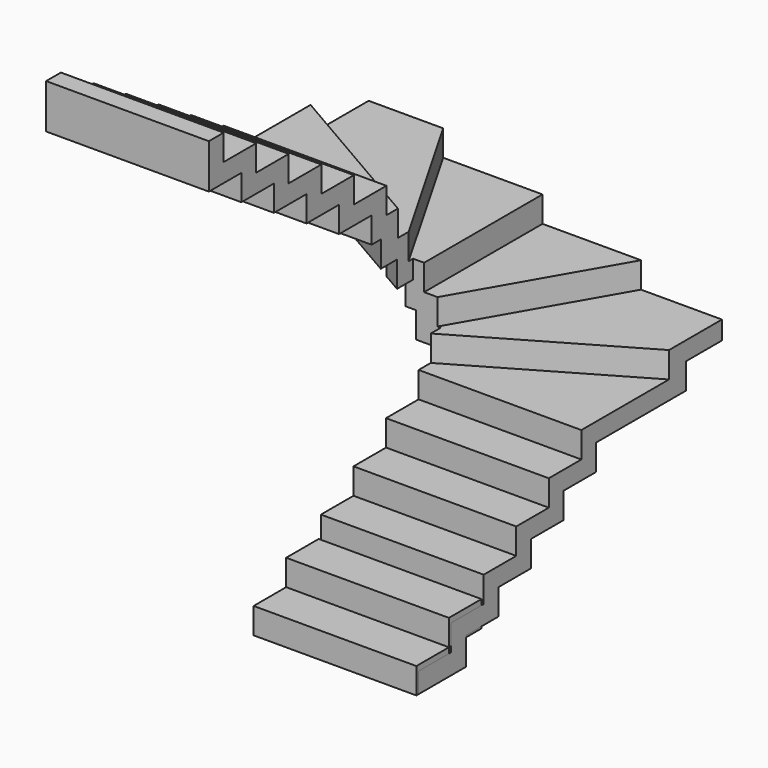
from build123d import *

# Parameters (mm, degrees)
F4_W           = 1117.6
F4_H           = 279.4
F6_DEPTH       = 177.8
F7_START       = 177.8
F7_DEPTH       = 177.8
F8_W           = 260.35
F8_H           = 139.7
F9_DEPTH       = 1117.6
F11_DEPTH      = 127
F12_DEPTH      = 177.8
F12_DEPTH_BACK = 127
F14_DEPTH      = 127
F15_DEPTH      = 177.8
F15_DEPTH_BACK = 127
F17_DEPTH      = 127
F18_DEPTH      = 177.8
F18_DEPTH_BACK = 127
F20_DEPTH      = 127
F21_DEPTH      = 177.8
F21_DEPTH_BACK = 127
F23_DEPTH      = 127
F24_DEPTH      = 177.8
F24_DEPTH_BACK = 127
F26_DEPTH      = 127
F27_DEPTH      = 177.8
F27_DEPTH_BACK = 127
F29_DEPTH      = 1117.6
F31_DEPTH      = 177.8


# Not quite as in the source:
# - a variable given as a bare number and used for a length is read in inches; the dataset says mm whatever the document's units were
# - a feature names something its author has since deleted; it is built from what else it names


with BuildPart() as f6:
    # F4 (on Top) → F6 (new body)
    with BuildSketch(Plane.XY):
        with Locations((654.05, -1257.3)):
            Rectangle(F4_W, F4_H)
    extrude(amount=F6_DEPTH)


with BuildPart() as f7:
    # F4 (on Top) → F7 (new body)
    with BuildSketch(Plane.XY.offset(F7_START)):
        with Locations((654.05, -977.9)):
            Rectangle(F4_W, F4_H)
    extrude(amount=F7_DEPTH)


with BuildPart() as f9:
    # F8 (on face) → F9 (new body)
    with BuildSketch(Plane.YZ.offset(1212.85)):
        Polygon((-1098.55, 139.7), (-1117.6, 139.7), (-1117.6, 0), (-971.55, 0), (-971.55, 190.5), (-692.15, 190.5), (-692.15, 368.3), (-412.75, 368.3), (-412.75, 546.1), (-133.35, 546.1), (-133.35, 723.9), (146.05, 723.9), (146.05, 1028.7), (19.05, 1028.7), (19.05, 850.9), (-260.35, 850.9), (-260.35, 673.1), (-539.75, 673.1), (-539.75, 495.3), (-819.15, 495.3), (-819.15, 317.5), (-1098.55, 317.5), align=None)
        with Locations((-1247.775, 69.85)):
            Rectangle(F8_W, F8_H)
    extrude(amount=-F9_DEPTH)

    # F10 (on face) → F11 (join)
    with BuildSketch(Plane.XY.offset(1028.7)):
        Polygon((1212.85, 771.3179841809), (133.9562233742, 146.05), (1212.85, 146.05), align=None)
    extrude(amount=-F11_DEPTH)

    # F10 (on face) → F12 (join, two sides)
    with BuildSketch(Plane.XY.offset(1028.7)) as f12_sk:
        Polygon((95.25, 146.05), (133.9562233742, 146.05), (1212.85, 771.3179841809), (1212.85, 918.1045453867), (-9.7539214515, 209.55), (95.25, 209.55), align=None)
        Polygon((95.25, 146.05), (95.25, 123.6179841809), (133.9562233742, 146.05), align=None)
    extrude(amount=F12_DEPTH)
    extrude(f12_sk.sketch, amount=-F12_DEPTH_BACK)

    # F13 (on face) → F14 (join)
    with BuildSketch(Plane.XY.offset(1206.5)):
        Polygon((1212.85, 1225.55), (657.4753068494, 1225.55), (114.7722326257, 281.7185665675), (1212.85, 918.1045453867), align=None)
    extrude(amount=-F14_DEPTH)

    # F13 (on face) → F15 (join, two sides)
    with BuildSketch(Plane.XY.offset(1206.5)) as f15_sk:
        Polygon((657.4753068494, 1225.55), (510.9773525122, 1225.55), (-73.2226474878, 209.55), (-9.7539214515, 209.55), (114.7722326257, 281.7185665675), align=None)
        Polygon((114.7722326257, 281.7185665675), (-9.7539214515, 209.55), (73.2753068494, 209.55), align=None)
    extrude(amount=F15_DEPTH)
    extrude(f15_sk.sketch, amount=-F15_DEPTH_BACK)

    # F16 (on face) → F17 (join)
    with BuildSketch(Plane.XY.offset(1384.3)):
        Polygon((510.9773525122, 1225.55), (-19.05, 1225.55), (-19.05, 303.7632999789), align=None)
    extrude(amount=-F17_DEPTH)

    # F16 (on face) → F18 (join, two sides)
    with BuildSketch(Plane.XY.offset(1384.3)) as f18_sk:
        Polygon((-19.05, 1225.55), (-146.05, 1225.55), (-146.05, 209.55), (-73.2226474878, 209.55), (-19.05, 303.7632999789), align=None)
        Polygon((-19.05, 303.7632999789), (-73.2226474878, 209.55), (-19.05, 209.55), align=None)
    extrude(amount=F18_DEPTH)
    extrude(f18_sk.sketch, amount=-F18_DEPTH_BACK)

    # F19 (on face) → F20 (join)
    with BuildSketch(Plane.XY.offset(1562.1)):
        Polygon((-146.05, 1225.55), (-701.4246931506, 1225.55), (-146.05, 259.6809684338), align=None)
        Polygon((-95.25, 209.55), (-117.2246931506, 209.55), (-95.25, 171.3331423468), align=None)
    extrude(amount=-F20_DEPTH)

    # F19 (on face) → F21 (join, two sides)
    with BuildSketch(Plane.XY.offset(1562.1)) as f21_sk:
        Polygon((-146.05, 259.6809684338), (-701.4246931506, 1225.55), (-847.9226474878, 1225.55), (-229.5123430682, 150.0538184006), (-95.25, 72.2426877588), (-95.25, 171.3331423468), (-117.2246931506, 209.55), (-146.05, 209.55), align=None)
        Polygon((-117.2246931506, 209.55), (-146.05, 259.6809684338), (-146.05, 209.55), align=None)
    extrude(amount=F21_DEPTH)
    extrude(f21_sk.sketch, amount=-F21_DEPTH_BACK)

    # F22 (on face) → F23 (join)
    with BuildSketch(Plane.XY.offset(1739.9)):
        Polygon((-235.841614476, 161.0612469359), (-847.9226474878, 1225.55), (-1212.85, 1225.55), (-1212.85, 727.2820158191), align=None)
    extrude(amount=-F23_DEPTH)

    # F22 (on face) → F24 (join, two sides)
    with BuildSketch(Plane.XY.offset(1739.9)) as f24_sk:
        Polygon((-229.5123430682, 150.0538184006), (-235.841614476, 161.0612469359), (-1212.85, 727.2820158191), (-1212.85, 580.4954546133), (-95.25, -67.2045453867), (-95.25, 72.2426877588), align=None)
        Polygon((-95.25, 79.5820158191), (-235.841614476, 161.0612469359), (-229.5123430682, 150.0538184006), (-95.25, 72.2426877588), align=None)
    extrude(amount=F24_DEPTH)
    extrude(f24_sk.sketch, amount=-F24_DEPTH_BACK)

    # F25 (on face) → F26 (join)
    with BuildSketch(Plane.XY.offset(1917.7)):
        Polygon((-178.3401959613, -19.05), (-1212.85, 580.4954546133), (-1212.85, -19.05), align=None)
    extrude(amount=-F26_DEPTH)

    # F25 (on face) → F27 (join, two sides)
    with BuildSketch(Plane.XY.offset(1917.7)) as f27_sk:
        Polygon((-178.3401959613, -19.05), (-1212.85, -19.05), (-1212.85, -146.05), (-95.25, -146.05), (-95.25, -67.2045453867), align=None)
        Polygon((-95.25, -19.05), (-178.3401959613, -19.05), (-95.25, -67.2045453867), align=None)
    extrude(amount=F27_DEPTH)
    extrude(f27_sk.sketch, amount=-F27_DEPTH_BACK)

    # F28 (on face) → F29 (join)
    with BuildSketch(Plane.YZ.offset(-95.25)):
        Polygon((-146.05, 1968.5), (-146.05, 2095.5), (-298.45, 2095.5), (-298.45, 2273.3), (-577.85, 2273.3), (-577.85, 2451.1), (-857.25, 2451.1), (-857.25, 2628.9), (-1136.65, 2628.9), (-1136.65, 2806.7), (-1416.05, 2806.7), (-1416.05, 2984.5), (-1543.05, 2984.5), (-1543.05, 2679.7), (-1263.65, 2679.7), (-1263.65, 2501.9), (-984.25, 2501.9), (-984.25, 2324.1), (-704.85, 2324.1), (-704.85, 2146.3), (-425.45, 2146.3), (-425.45, 1968.5), align=None)
    extrude(amount=-F29_DEPTH)

    # F30 (on face) → F31 (cut)
    with BuildSketch(Plane(origin=(0, 0, 901.7), x_dir=(1, 0, 0), z_dir=(0, 0, -1))):
        Polygon((95.25, -270.4045453867), (95.25, -209.55), (-9.7539214515, -209.55), align=None)
    extrude(amount=-F31_DEPTH, mode=Mode.SUBTRACT)


solid = Compound([f6.part, f7.part, f9.part])
